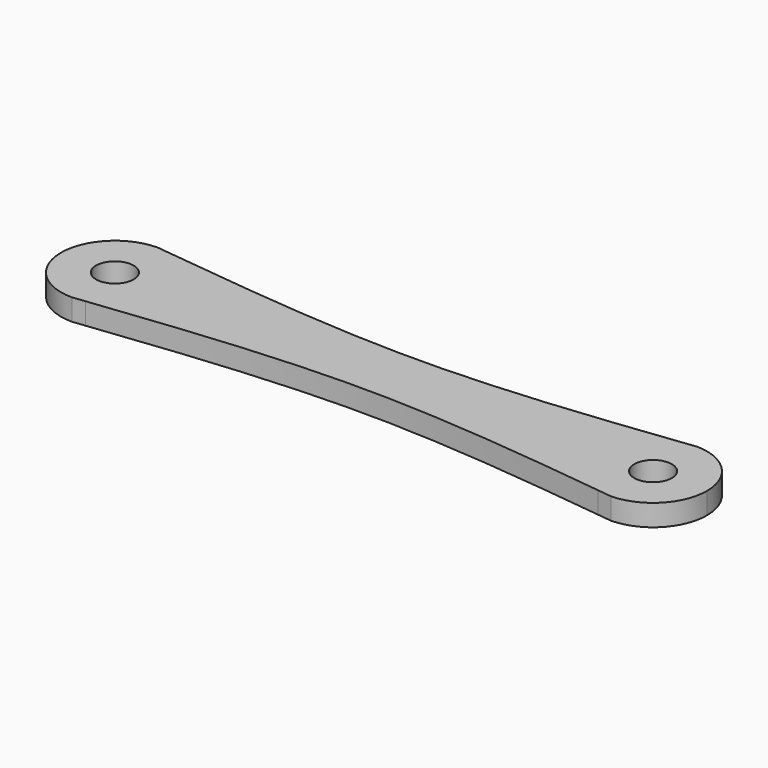
from build123d import *

# Parameters (mm, degrees)
F0_R     = 1.75
F1_DEPTH = 2


with BuildPart() as f1:
    # F0 (on Top) → F1 (new body)
    with BuildSketch(Plane.XY):
        with BuildLine():
            add(Edge.make_bspline(
                [(0, 5), (0.3879096976, 4.9541997763), (0.7758195621, 4.9083974868), (1.1637210766, 4.8626899198)],
                knots=[0, 0, 0, 0, 0.0229747267, 0.0229747267, 0.0229747267, 0.0229747267], degree=3))
            ThreePointArc((0, 5), (-5, 0), (0, -5))
            add(Edge.make_bspline(
                [(0, -5), (0.3884219151, -4.9540765878), (0.7768439434, -4.9081517555), (1.1652569528, -4.8623221031)],
                knots=[0, 0, 0, 0, 0.0230119064, 0.0230119064, 0.0230119064, 0.0230119064], degree=3))
            ThreePointArc((1.1652569528, -4.8623221031), (3.9259575115, -3.0962651078), (5, 0))
            ThreePointArc((5, 0), (3.9254684678, 3.0968850977), (1.1637210766, 4.8626899198))
        make_face()
        Circle(F0_R, mode=Mode.SUBTRACT)
        with BuildLine():
            add(Edge.make_bspline(
                [(1.1637210766, 4.8626899198), (9.2762111087, 3.9067715533), (25.2735349116, 2.1026460012), (40.9534234423, 3.9056306073), (48.6808792271, 4.8436985253)],
                knots=[0.0229747267, 0.0229747267, 0.0229747267, 0.0229747267, 0.5034632902, 0.9708949207, 0.9708949207, 0.9708949207, 0.9708949207], degree=3))
            ThreePointArc((1.1637210766, 4.8626899198), (3.9254684678, 3.0968850977), (5, 0))
            ThreePointArc((5, 0), (3.9259575115, -3.0962651078), (1.1652569528, -4.8623221031))
            add(Edge.make_bspline(
                [(1.1652569528, -4.8623221031), (9.2793010918, -3.9049292925), (25.3078629948, -2.0948602578), (40.9958544704, -3.8869187833), (48.7415823678, -4.8182057098)],
                knots=[0.0230119064, 0.0230119064, 0.0230119064, 0.0230119064, 0.5037363411, 0.9731005035, 0.9731005035, 0.9731005035, 0.9731005035], degree=3))
            ThreePointArc((48.7415823678, -4.8182057098), (45.0000943344, -0.0105696626), (48.6808792271, 4.8436985253))
        make_face()
        with BuildLine():
            add(Edge.make_bspline(
                [(48.6808792271, 4.8436985253), (49.1620366811, 4.9021082249), (49.6431766931, 4.9607078729), (50.1243168109, 5.0192975561)],
                knots=[0.9708949207, 0.9708949207, 0.9708949207, 0.9708949207, 1, 1, 1, 1], degree=3))
            ThreePointArc((48.6808792271, 4.8436985253), (45.0000943344, -0.0105696626), (48.7415823678, -4.8182057098))
            add(Edge.make_bspline(
                [(48.7415823678, -4.8182057098), (49.1854939332, -4.8715782324), (49.629390795, -4.9251017483), (50.0732877564, -4.9786194279)],
                knots=[0.9731005035, 0.9731005035, 0.9731005035, 0.9731005035, 1, 1, 1, 1], degree=3))
            ThreePointArc((50.0732877564, -4.9786194279), (53.5613479622, -3.488682203), (54.9999956555, 0.02084337))
            ThreePointArc((54.9999956555, 0.02084337), (53.5792138507, 3.5121464379), (50.1243168109, 5.0192975561))
        make_face()
        with Locations((49.9999956555, 0.02084337)):
            Circle(F0_R, mode=Mode.SUBTRACT)
    extrude(amount=F1_DEPTH)


solid = f1.part
